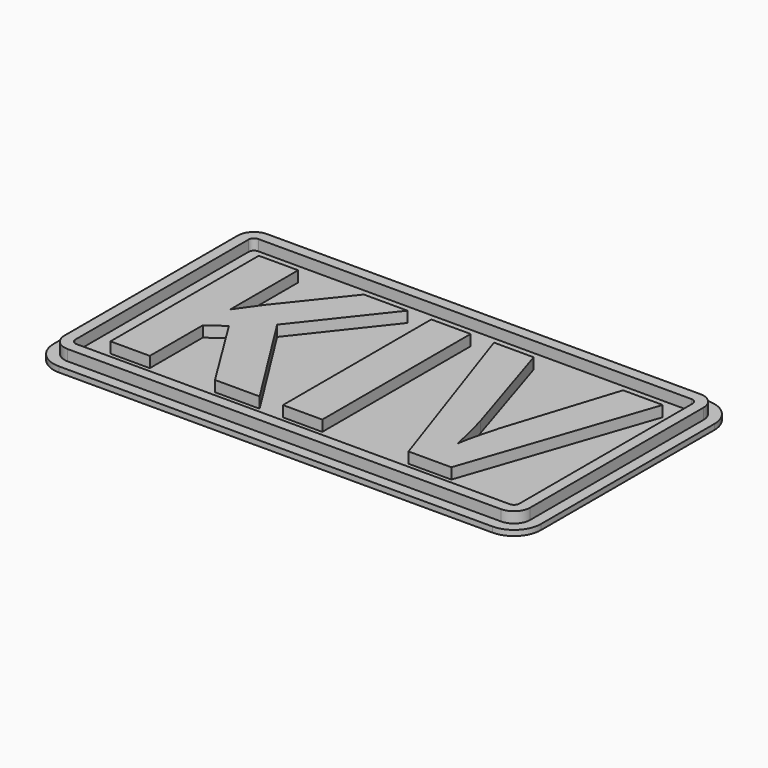
from build123d import *

# Parameters (mm, degrees)
F3_DEPTH     = 1
F4_TEXT_SIZE = 47.9575984648
F5_DEPTH     = 2


# Not quite as in the source:
# - Text() gives the source's letters only with a copy of the font that has no kerning and outlines rounded to 1/6400 em; it was checked with that copy


with BuildPart() as f3:
    # F2 (on Top) → F3 (new body)
    with BuildSketch(Plane.XY):
        with BuildLine():
            Line((40, 25), (-40, 25))
            ThreePointArc((-40, 25), (-43.5355339059, 23.5355339059), (-45, 20))
            Line((-45, 20), (-45, -20))
            ThreePointArc((-45, -20), (-43.5355339059, -23.5355339059), (-40, -25))
            Line((-40, -25), (40, -25))
            ThreePointArc((40, -25), (43.5355339059, -23.5355339059), (45, -20))
            Line((45, -20), (45, 20))
            ThreePointArc((45, 20), (43.5355339059, 23.5355339059), (40, 25))
        make_face()
    extrude(amount=F3_DEPTH)

    # F4 (on face) → F5 (join)
    with BuildSketch(Plane.XY.offset(1)):
        with BuildLine():
            Line((40, 23), (-40, 23))
            ThreePointArc((-40, 23), (-42.1213203436, 22.1213203436), (-43, 20))
            Line((-43, 20), (-43, -20))
            ThreePointArc((-43, -20), (-42.1213203436, -22.1213203436), (-40, -23))
            Line((-40, -23), (40, -23))
            ThreePointArc((40, -23), (42.1213203436, -22.1213203436), (43, -20))
            Line((43, -20), (43, 20))
            ThreePointArc((43, 20), (42.1213203436, 22.1213203436), (40, 23))
        make_face()
        with BuildLine():
            ThreePointArc((-41, 20), (-40.7071067812, 20.7071067812), (-40, 21))
            Line((-40, 21), (40, 21))
            ThreePointArc((40, 21), (40.7071067812, 20.7071067812), (41, 20))
            Line((41, 20), (41, -20))
            ThreePointArc((41, -20), (40.7071067812, -20.7071067812), (40, -21))
            Line((40, -21), (-40, -21))
            ThreePointArc((-40, -21), (-40.7071067812, -20.7071067812), (-41, -20))
            Line((-41, -20), (-41, 20))
        make_face(mode=Mode.SUBTRACT)
        with Locations((-41, -17.2647354473)):
            Text('KIV', F4_TEXT_SIZE, font='Open Sans', font_style=FontStyle.BOLD, text_align=(TextAlign.LEFT, TextAlign.BOTTOM))
    extrude(amount=F5_DEPTH)


solid = f3.part
